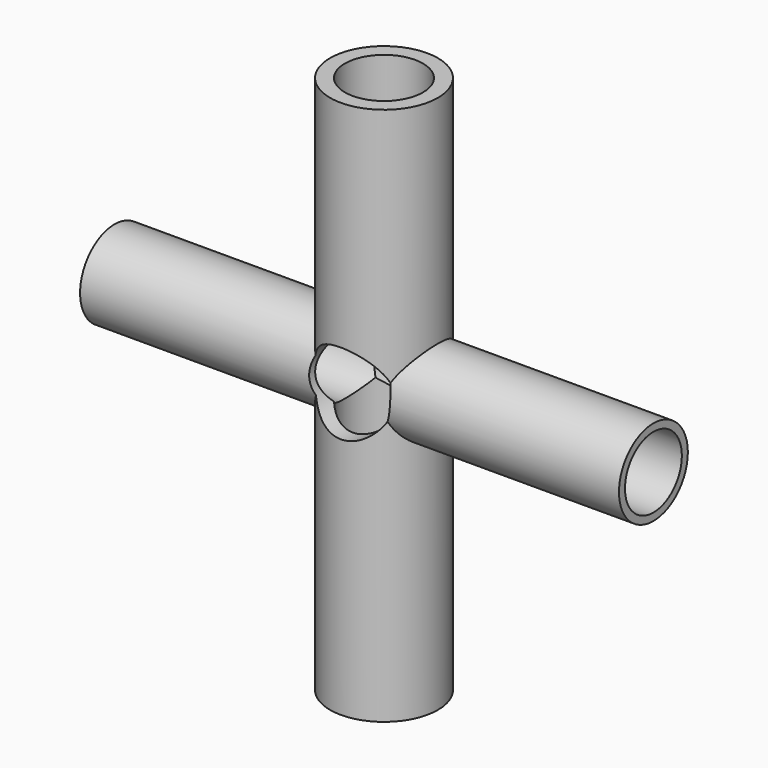
from build123d import *

# Parameters (mm, degrees)
F0_R      = 2.5
F1_DEPTH  = 25
F3_R      = 1.996994491
F4_DEPTH  = 12.5
F5_R      = 1.6492886798
F6_DEPTH  = 12
F2_R      = 1.8125623044
F7_DEPTH  = 25.0010001
F8_R      = 1.8761766921
F9_DEPTH  = 2.5010001
F10_DEPTH = 2.5010001


# Not quite as in the source:
# - a pattern or mirror of a feature is missing from the dataset's text; its kind, count and spacing are read off the source's solid


with BuildPart() as f1:
    # F0 (on Top) → F1 (new body)
    with BuildSketch(Plane.XY):
        Circle(F0_R)
    extrude(amount=F1_DEPTH)

    # F3 (on Right) → F4 (join)
    with BuildSketch(Plane.YZ):
        with Locations((0, 12.9643771797)):
            Circle(F3_R)
    f4 = extrude(amount=F4_DEPTH)

    # F4_copies: F4 across plane
    add(f4.mirror(Plane(origin=(1.1e-05, 0, 0), x_dir=(0, 0, -1), z_dir=(-1, 0, 0))))

    # F5 (on face) → F6 (cut)
    with BuildSketch(Plane.YZ.offset(12.5)):
        with Locations((0, 12.9643771797)):
            Circle(F5_R)
    f6 = extrude(amount=-F6_DEPTH, mode=Mode.SUBTRACT)

    # F6_copies: F6 across plane
    add(f6.mirror(Plane(origin=(1e-05, 0, 0), x_dir=(0, 0, -1), z_dir=(-1, 0, 0))), mode=Mode.SUBTRACT)

    # F2 (on face) → F7 (cut, through all)
    with BuildSketch(Plane.XY.offset(25)):
        Circle(F2_R)
    extrude(amount=-F7_DEPTH, mode=Mode.SUBTRACT)

    # F8 (on Front) → F9 (cut, through all)
    with BuildSketch(Plane.XZ):
        with Locations((0, 13.1307579577)):
            Circle(F8_R)
    extrude(amount=F9_DEPTH, mode=Mode.SUBTRACT)

    # F8 (on Front) → F10 (cut, through all)
    with BuildSketch(Plane.XZ):
        with Locations((0, 13.1307579577)):
            Circle(F8_R)
    extrude(amount=-F10_DEPTH, mode=Mode.SUBTRACT)


solid = f1.part
